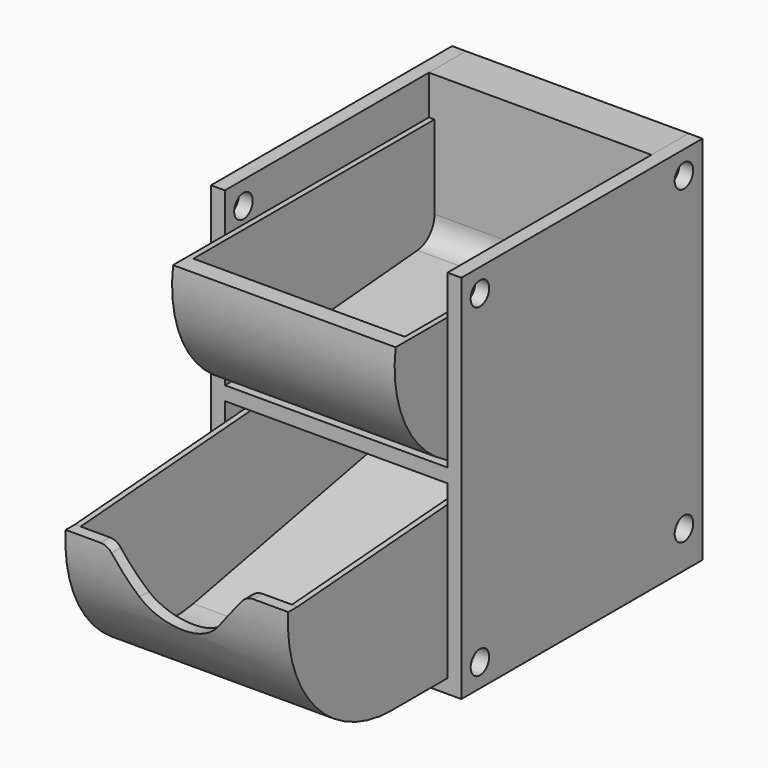
from build123d import *

# Parameters (mm, degrees)
F1_DEPTH  = 80
F2_W      = 48
F2_H      = 37
F3_DEPTH  = 65.001
F4_DEPTH  = 11.8
F5_W      = 48
F5_H      = 3
F6_DEPTH  = 15
F7_DEPTH  = 11.8
F8_W      = 48
F8_H      = 1.5
F9_DEPTH  = 15
F11_DEPTH = 24
F12_R     = 2.5
F13_DEPTH = 30
F15_DEPTH = 43.001
F16_R     = 3.1
F18_DEPTH = 1.2
F20_DEPTH = 1.2
F22_DEPTH = 24
F24_DEPTH = 1.2
F26_DEPTH = 1.2


# Not quite as in the source:
# - a feature names something its author has since deleted; it is built from what else it names


with BuildPart() as f1:
    # F0 (on Top) → F1 (new body)
    with BuildSketch(Plane.XY):
        Polygon((-24, 65), (-27, 65), (-27, 0), (27, 0), (27, 65), (24, 65), (24, 3), (-24, 3), align=None)
    extrude(amount=F1_DEPTH)

    # F2 (on face) → F3 (cut, through all)
    with BuildSketch(Plane.XZ):
        with Locations((0, 21.5)):
            Rectangle(F2_W, F2_H)
        with Locations((0, 61.5)):
            Rectangle(F2_W, F2_H)
    extrude(amount=-F3_DEPTH, mode=Mode.SUBTRACT)

    # F4 (add): a face of the model
    f4_faces = [f1.faces().sort_by_distance(p)[0] for p in [
        (0, 3, 1.5),
    ]]
    extrude(f4_faces, amount=F4_DEPTH)

    # F5 (on face) → F6 (join)
    with BuildSketch(Plane(origin=(0, 65, 0), x_dir=(-1, 0, 0), z_dir=(0, 1, 0))):
        with Locations((0, 1.5)):
            Rectangle(F5_W, F5_H)
    extrude(amount=-F6_DEPTH)

    # F7 (add, through all): a face of the model
    f7_faces = [f1.faces().sort_by_distance(p)[0] for p in [
        (0, 3, 41.5),
    ]]
    extrude(f7_faces, amount=F7_DEPTH)

    # F8 (on face) → F9 (join)
    with BuildSketch(Plane(origin=(0, 65, 0), x_dir=(-1, 0, 0), z_dir=(0, 1, 0))):
        with Locations((0, 40.75)):
            Rectangle(F8_W, F8_H)
    extrude(amount=-F9_DEPTH)


with BuildPart() as f11:
    # F10 (on Right) → F11 (new body, symmetric)
    with BuildSketch(Plane.YZ):
        with BuildLine():
            Line((65, 3), (65, 21))
            Line((65, 21), (65, 40))
            Line((65, 40), (55, 40))
            Line((55, 40), (55, 23.0990195136))
            ThreePointArc((55, 23.0990195136), (53.8667107067, 19.9290749856), (50.9805806757, 18.1961161351))
            Line((50.9805806757, 18.1961161351), (-10, 6))
            ThreePointArc((-10, 6), (-31.9250900991, 11.9332403084), (-40.4165300543, 33))
            Line((-40.4165300543, 33), (-42.9284800875, 33))
            ThreePointArc((-42.9284800875, 33), (-35.4939015319, 11.9212159717), (-15, 3))
            Line((-15, 3), (55, 3))
            Line((55, 3), (65, 3))
        make_face()
    extrude(amount=F11_DEPTH, both=True)


with BuildPart() as f13_tool:
    # F12 (on Right) → F13 (new body, symmetric)
    with BuildSketch(Plane.YZ):
        with Locations((60, 75)):
            Circle(F12_R)
        with Locations((60, 8)):
            Circle(F12_R)
        with Locations((5, 75)):
            Circle(F12_R)
        with Locations((5, 5)):
            Circle(F12_R)
    extrude(amount=F13_DEPTH, both=True)


with BuildPart() as f1_1:
    add(f1.part)

    # F13: cut by f13_tool
    add(f13_tool.part, mode=Mode.SUBTRACT)


with BuildPart() as f11_1:
    add(f11.part)

    # F13: cut by f13_tool
    add(f13_tool.part, mode=Mode.SUBTRACT)

    # F14 (on Front) → F15 (cut, through all)
    with BuildSketch(Plane.XZ):
        with BuildLine():
            Line((-15, 33), (-8.5297188426, 25.0542173611))
            ThreePointArc((-8.5297188426, 25.0542173611), (0, 21), (8.5297188426, 25.0542173611))
            Line((8.5297188426, 25.0542173611), (15, 33))
            Line((15, 33), (-15, 33))
        make_face()
    extrude(amount=F15_DEPTH, mode=Mode.SUBTRACT)

    # F16
    f16_edges = [f11_1.edges().sort_by_distance(p)[0] for p in [
        (-15, -41.672505, 33),
        (15, -41.672505, 33),
    ]]
    fillet(f16_edges, radius=F16_R)

    # F17 (on face) → F18 (join)
    with BuildSketch(Plane.YZ.offset(24)):
        with BuildLine():
            ThreePointArc((-40.4165300543, 33), (-31.9250900991, 11.9332403084), (-10, 6))
            Line((-10, 6), (50.9805806757, 18.1961161351))
            ThreePointArc((50.9805806757, 18.1961161351), (53.8667107067, 19.9290749856), (55, 23.0990195136))
            Line((55, 23.0990195136), (55, 40))
            Line((55, 40), (-40.4165300543, 33))
        make_face()
    extrude(amount=-F18_DEPTH)

    # F19 (on face) → F20 (join)
    with BuildSketch(Plane(origin=(-24, 0, 0), x_dir=(0, -1, 0), z_dir=(-1, 0, 0))):
        with BuildLine():
            ThreePointArc((-55, 23.0990195136), (-53.8667107067, 19.9290749856), (-50.9805806757, 18.1961161351))
            Line((-50.9805806757, 18.1961161351), (10, 6))
            ThreePointArc((10, 6), (31.9250900991, 11.9332403084), (40.4165300543, 33))
            Line((40.4165300543, 33), (-55, 40))
            Line((-55, 40), (-55, 23.0990195136))
        make_face()
    extrude(amount=-F20_DEPTH)


with BuildPart() as f22:
    # F21 (on Right) → F22 (new body, symmetric)
    with BuildSketch(Plane.YZ):
        with BuildLine():
            Line((65, 80), (55, 80))
            Line((55, 80), (55, 53.5))
            ThreePointArc((55, 53.5), (53.677981268, 50.1128989103), (50.4110184832, 48.5169222556))
            Line((50.4110184832, 48.5169222556), (13.8346630084, 45.5))
            ThreePointArc((13.8346630084, 45.5), (-4.4517538274, 52.6613460558), (-10, 71.5))
            Line((-10, 71.5), (-13.9726337853, 71.5))
            ThreePointArc((-13.9726337853, 71.5), (-7.8404744509, 50.5659825278), (12, 41.5))
            Line((12, 41.5), (65, 41.5))
            Line((65, 41.5), (65, 80))
        make_face()
    extrude(amount=F22_DEPTH, both=True)

    # F23 (on face) → F24 (join)
    with BuildSketch(Plane.YZ.offset(24)):
        with BuildLine():
            Line((55, 71.5), (-10, 71.5))
            ThreePointArc((-10, 71.5), (-4.4517538274, 52.6613460558), (13.8346630084, 45.5))
            Line((13.8346630084, 45.5), (50.3340224507, 48.510571403))
            Line((50.3340224507, 48.510571403), (50.4110184832, 48.5169222556))
            ThreePointArc((50.4110184832, 48.5169222556), (53.677981268, 50.1128989103), (55, 53.5))
            Line((55, 53.5), (55, 71.5))
        make_face()
    extrude(amount=-F24_DEPTH)

    # F25 (on face) → F26 (join)
    with BuildSketch(Plane(origin=(-24, 0, 0), x_dir=(0, -1, 0), z_dir=(-1, 0, 0))):
        with BuildLine():
            ThreePointArc((-13.8346630084, 45.5), (4.4517538274, 52.6613460558), (10, 71.5))
            Line((10, 71.5), (-55, 71.5))
            Line((-55, 71.5), (-55, 53.5))
            ThreePointArc((-55, 53.5), (-53.677981268, 50.1128989103), (-50.4110184832, 48.5169222556))
            Line((-50.4110184832, 48.5169222556), (-13.8346630084, 45.5))
        make_face()
    extrude(amount=-F26_DEPTH)


solid = Compound([f1_1.part, f11_1.part, f22.part])
